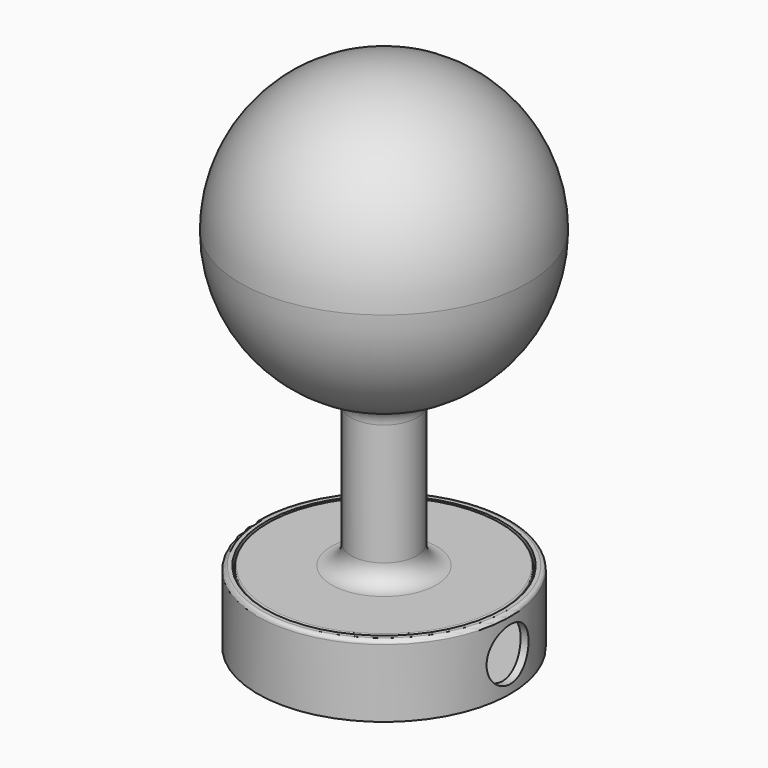
from build123d import *

# Parameters (mm, degrees)
F7_R     = 6.75
F8_DEPTH = 50


with BuildPart() as f2:
    # F0 (on Right) → F2 (revolve)
    with BuildSketch(Plane.YZ):
        with BuildLine():
            ThreePointArc((-8.5, -71), (-9.9644660941, -74.5355339059), (-13.5, -76))
            Line((-13.5, -76), (-29.6944898516, -76))
            ThreePointArc((-29.6944898516, -76), (-29.9105181493, -76.0894818507), (-30, -76.3055101484))
            Line((-30, -76.3055101484), (-30, -78))
            Line((-30, -78), (-6.5, -78))
            Line((-6.5, -78), (-6.5, -76))
            Line((-6.5, -76), (-6.5, -75))
            Line((-6.5, -75), (-6.5, -36.588932753))
            Line((-6.5, -36.588932753), (-6.5, -35.1541249358))
            ThreePointArc((-6.5, -35.1541249358), (-27.4812436036, -22.8657768291), (-35.75, 0))
            Line((-35.75, 0), (-37, 0))
            ThreePointArc((-37, 0), (-30.07520336, -21.5518477829), (-11.8928571429, -35.0365516137))
            ThreePointArc((-11.8928571429, -35.0365516137), (-9.4357833297, -36.8588088881), (-8.5, -39.7712207507))
            Line((-8.5, -39.7712207507), (-8.5, -71))
        make_face()
    revolve(axis=Axis((0, 0, -37.5008806586), (0, 0, 1)))


with BuildPart() as f4:
    # F3 (on Front) → F4 (revolve)
    with BuildSketch(Plane.XZ):
        with BuildLine():
            Line((0, 36), (0, 37))
            ThreePointArc((0, 37), (-26.1629509039, 26.1629509039), (-37, 0))
            Line((-37, 0), (-36, 0))
            ThreePointArc((-36, 0), (-25.4558441227, 25.4558441227), (0, 36))
        make_face()
    revolve(axis=Axis((0, 0, 36.5), (0, 0, 1)))

    # F9 (on Front) → F10 (revolve)
    with BuildSketch(Plane.XZ):
        with BuildLine():
            Line((-36.1092984676, 0), (-35.5, 0))
            ThreePointArc((-35.5, 0), (-35.4859014997, -1.0003972986), (-35.4436171969, -2))
            Line((-35.4436171969, -2), (-33.941125497, -2))
            ThreePointArc((-33.941125497, -2), (-33.9990784283, -0.2503318301), (-33.9668956486, 1.5))
            Line((-33.9668956486, 1.5), (-36.1092984676, 1.5))
            Line((-36.1092984676, 1.5), (-36.1092984676, 0))
        make_face()
    revolve(axis=Axis((0, 0, -37.5008806586), (0, 0, 1)))


with BuildPart() as f6:
    # F5 (on Right) → F6 (revolve)
    with BuildSketch(Plane.YZ):
        with BuildLine():
            Line((-30.5, -78.5151124001), (-30.5, -76))
            Line((-30.5, -76), (-31.5, -76))
            ThreePointArc((-31.5, -76), (-32.2071067812, -76.2928932188), (-32.5, -77))
            Line((-32.5, -77), (-32.5, -92.5151124001))
            Line((-32.5, -92.5151124001), (-32.5, -94.5151124001))
            Line((-32.5, -94.5151124001), (0, -94.5151124001))
            Line((0, -94.5151124001), (0, -92.5151124001))
            Line((0, -92.5151124001), (-30.5, -92.5151124001))
            Line((-30.5, -92.5151124001), (-30.5, -81.5151124001))
            ThreePointArc((-30.5, -81.5151124001), (-30.2071067812, -80.8080056189), (-29.5, -80.5151124001))
            Line((-29.5, -80.5151124001), (-28.5, -80.5151124001))
            Line((-28.5, -80.5151124001), (-28.5, -78.5151124001))
            Line((-28.5, -78.5151124001), (-30.5, -78.5151124001))
        make_face()
    revolve(axis=Axis((0, 0, -93.5151124001), (0, 0, 1)))

    # F7 (on Right) → F8 (cut)
    with BuildSketch(Plane.YZ):
        with Locations((0, -85.5151124001)):
            Circle(F7_R)
    extrude(amount=F8_DEPTH, mode=Mode.SUBTRACT)


solid = Compound([f2.part, f4.part, f6.part])
